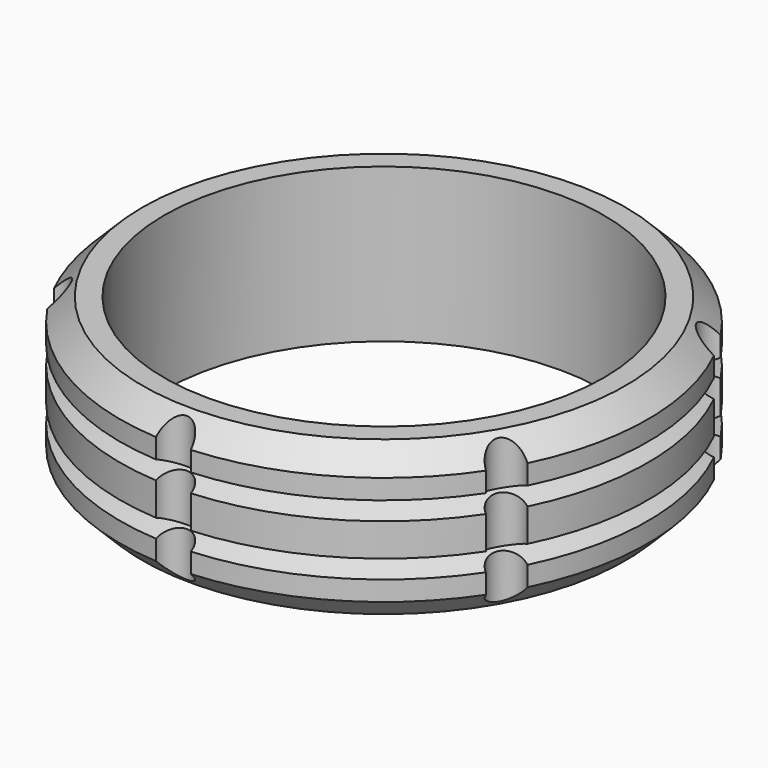
from build123d import *

# Parameters (mm, degrees)
F2_SIZE  = 1.016
F3_R     = 0.79375
F4_DEPTH = 7.001


with BuildPart() as f1:
    # F0 (on Front) → F1 (revolve)
    with BuildSketch(Plane.XZ):
        Polygon((-12, 0), (-10, 0), (-10, 7), (-12, 7), (-12, 5.085014044), (-11, 4.6666666667), (-12, 4.2483192893), (-12, 2.7516807107), (-11, 2.3333333333), (-12, 1.914985956), align=None)
    revolve(axis=Axis((0, 0, 5.7299032821), (0, 0, -1)))

    # F2
    f2_edges = [f1.edges().sort_by_distance(p)[0] for p in [
        (12, 0, 7),
        (12, 0, 0),
    ]]
    chamfer(f2_edges, length=F2_SIZE)

    # F3 (on Top) → F4 (cut, through all)
    with BuildSketch(Plane.XY):
        with Locations((-10.3923048454, -6)):
            Circle(F3_R)
        with Locations((0, -12)):
            Circle(F3_R)
        with Locations((10.3923048454, -6)):
            Circle(F3_R)
        with Locations((10.3923048454, 6)):
            Circle(F3_R)
        with Locations((0, 12)):
            Circle(F3_R)
        with Locations((-10.3923048454, 6)):
            Circle(F3_R)
    extrude(amount=F4_DEPTH, mode=Mode.SUBTRACT)


solid = f1.part
